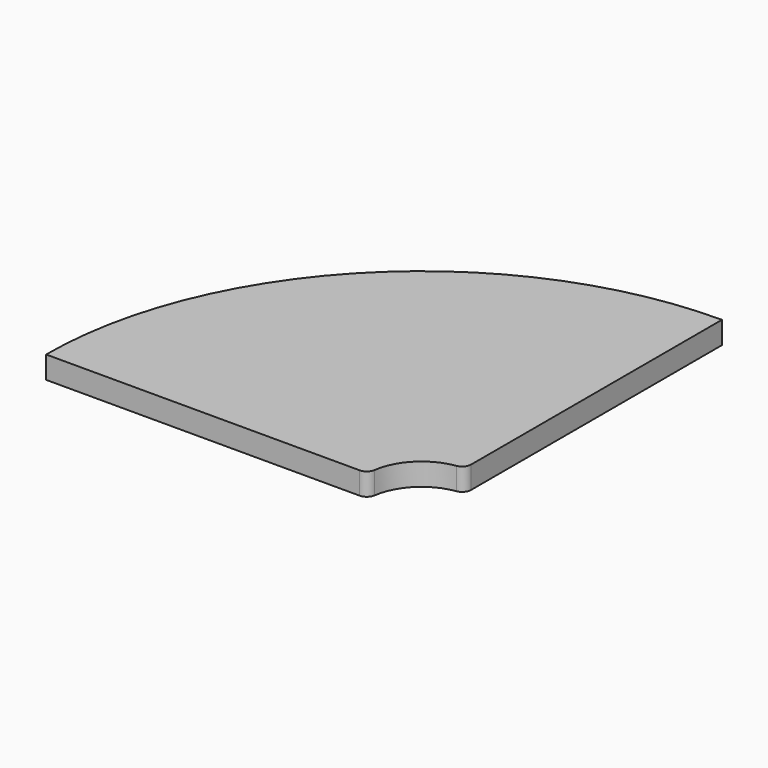
from build123d import *

# Parameters (mm, degrees)
F1_DEPTH = 3.175
F2_R     = 1.27


# Not quite as in the source:
# - a feature names something its author has since deleted; it is built from what else it names


with BuildPart() as f1:
    # F0 (on Top) → F1 (new body)
    with BuildSketch(Plane.XY):
        with BuildLine():
            Line((0, 7.62), (0, 12.7))
            ThreePointArc((0, 12.7), (-8.9802561211, 8.9802561211), (-12.7, 0))
            Line((-12.7, 0), (-7.62, 0))
            ThreePointArc((-7.62, 0), (-5.3881536726, 5.3881536726), (0, 7.62))
        make_face()
        with BuildLine():
            ThreePointArc((-12.7, 0), (-8.9802561211, 8.9802561211), (0, 12.7))
            Line((0, 12.7), (0, 48.26))
            ThreePointArc((0, 48.26), (-34.1249732601, 34.1249732601), (-48.26, 0))
            Line((-48.26, 0), (-12.7, 0))
        make_face()
        with BuildLine():
            ThreePointArc((-48.26, 0), (-34.1249732601, 34.1249732601), (0, 48.26))
            Line((0, 48.26), (0, 53.34))
            ThreePointArc((0, 53.34), (-37.7170757085, 37.7170757085), (-53.34, 0))
            Line((-53.34, 0), (-48.26, 0))
        make_face()
    extrude(amount=F1_DEPTH)

    # F2
    f2_edges = [f1.edges().sort_by_distance(p)[0] for p in [
        (-7.62, 0, 1.5875),
        (0, 7.62, 1.5875),
    ]]
    fillet(f2_edges, radius=F2_R)


solid = f1.part
